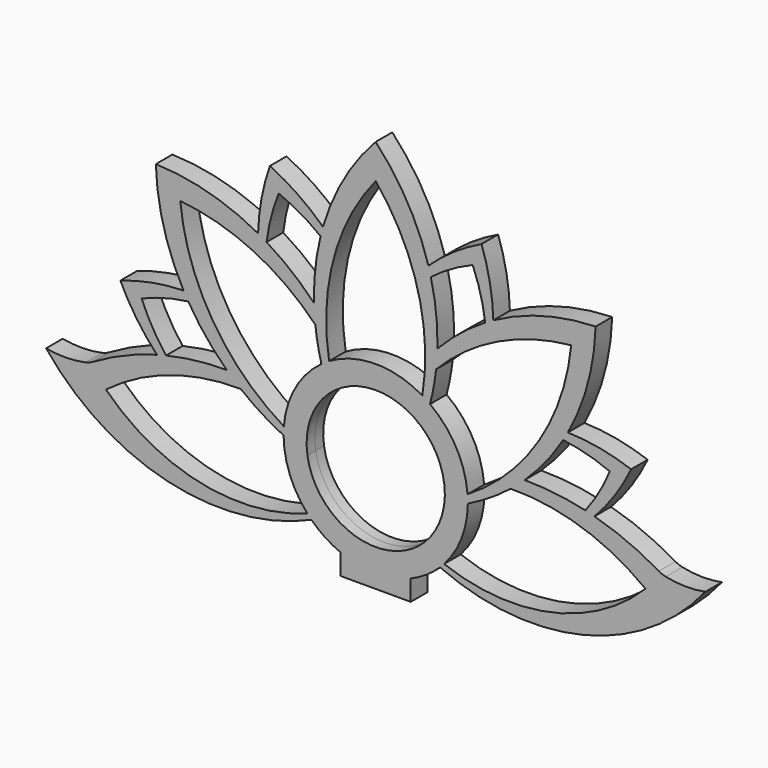
from build123d import *

# Parameters (mm, degrees)
F1_DEPTH = 4.5


# Not quite as in the source:
# - ends of sketch curves that miss each other by under 0.0002 mm in the source are joined


with BuildPart() as f1:
    # F0 (on Front) → F1 (new body, symmetric)
    with BuildSketch(Plane.XZ):
        with BuildLine():
            ThreePointArc((22.8784841202, 85.4427339913), (13.8060493669, 106.7545909747), (-1.20352e-05, 125.3528970532))
            ThreePointArc((-1.20352e-05, 125.3528970532), (-13.8060738367, 106.7545832167), (-22.8785085989, 85.4427260857))
            ThreePointArc((-22.8785085989, 85.4427260857), (-33.781429845, 94.2345199978), (-45.9220242093, 101.2184408782))
            ThreePointArc((-45.9220242093, 101.2184408782), (-49.5683429395, 87.6953665193), (-51.06114092, 73.7691058897))
            ThreePointArc((-51.06114092, 73.7691058897), (-72.5460800364, 82.4236845525), (-95.4594281867, 85.8123133595))
            ThreePointArc((-95.4594281867, 85.8123133595), (-92.0708001004, 62.8989646397), (-83.4162216453, 41.4140256538))
            ThreePointArc((-83.4162216453, 41.4140256538), (-97.3424818216, 39.9212276371), (-110.8655561911, 36.2749088727))
            ThreePointArc((-110.8655561911, 36.2749088727), (-103.8306945008, 24.0599857757), (-94.9659655862, 13.1005055314))
            ThreePointArc((-94.9659655862, 13.1005055314), (-109.3441086085, 8.1228594383), (-122.9337436667, 1.2796299938))
            ThreePointArc((-122.9337436667, 1.2796299938), (-124.3847743538, 0.5744976537), (-125.9303092338, 0.1118710562))
            ThreePointArc((-125.9303092338, 0.1118710562), (-134.5040813307, -0.8405705466), (-143.0970012567, -0.0800174007))
            ThreePointArc((-143.0970012567, -0.0800174007), (-90.2945054943, -33.7590284811), (-27.9154142382, -28.1707970164))
            ThreePointArc((-27.9154142382, -28.1707970164), (-21.9577774473, -32.956766848), (-15.1986970778, -36.5224048048))
            Line((-15.1986970778, -36.5224048048), (-15.1986972, -45.5224051023))
            Line((-15.1986972, -45.5224051023), (15.1986718, -45.5224051023))
            Line((15.1986718, -45.5224051023), (15.1986718, -36.5224051023))
            ThreePointArc((15.1986718, -36.5224051023), (21.9577523614, -32.9567672985), (27.9153889991, -28.1707973067))
            ThreePointArc((27.9153889991, -28.1707973067), (90.2944800943, -33.7590284811), (143.096975735, -0.0800170504))
            ThreePointArc((143.096975735, -0.0800170504), (134.5040559307, -0.8405705466), (125.9302837161, 0.1118705041))
            ThreePointArc((125.9302837161, 0.1118705041), (124.3847489538, 0.5744976537), (122.9337187314, 1.2796307814))
            ThreePointArc((122.9337187314, 1.2796307814), (109.3440836528, 8.1228592505), (94.9659404823, 13.1005047349))
            ThreePointArc((94.9659404823, 13.1005047349), (103.8306699794, 24.0599855987), (110.8655315962, 36.2749085192))
            ThreePointArc((110.8655315962, 36.2749085192), (97.3424564216, 39.9212276371), (83.416195792, 41.4140256177))
            ThreePointArc((83.416195792, 41.4140256177), (92.0707747004, 62.8989646397), (95.4594032906, 85.8123128836))
            ThreePointArc((95.4594032906, 85.8123128836), (72.5460546364, 82.4236845525), (51.0611157869, 73.7691059217))
            ThreePointArc((51.0611157869, 73.7691059217), (49.568318506, 87.695366698), (45.9219996628, 101.2184412045))
            ThreePointArc((45.9219996628, 101.2184412045), (33.7814018374, 94.2345137024), (22.8784841202, 85.4427339913))
        make_face()
        with BuildLine():
            ThreePointArc((-117.1095228717, -7.3640305351), (-89.448563488, 7.1418522166), (-58.5697361978, 11.837311045))
            ThreePointArc((-58.5697361978, 11.837311045), (-49.6119110254, 5.4631464022), (-39.9984925953, 0.1288430808))
            ThreePointArc((-39.9984925953, 0.1288430808), (-37.2748571799, -14.0339843315), (-29.705402075, -26.3102719896))
            ThreePointArc((-29.705402075, -26.3102719896), (-76.1944797379, -29.6944118928), (-117.1095228717, -7.3640305351))
        make_face(mode=Mode.SUBTRACT)
        with BuildLine():
            ThreePointArc((-91.0135912807, 14.1048128348), (-96.9513599422, 22.91124928), (-101.6267610462, 32.4480749604))
            ThreePointArc((-101.6267610462, 32.4480749604), (-91.6920273332, 35.8548732281), (-81.3873643524, 37.8844380956))
            ThreePointArc((-81.3873643524, 37.8844380956), (-73.7352473768, 26.9438563456), (-64.6715808547, 17.1407372042))
            ThreePointArc((-64.6715808547, 17.1407372042), (-77.9309186705, 16.3892197846), (-91.0135912807, 14.1048128348))
        make_face(mode=Mode.SUBTRACT)
        with BuildLine():
            ThreePointArc((-39.8747349061, 3.6409013815), (-70.812382671, 34.1134059196), (-84.8528261577, 75.2057109018))
            ThreePointArc((-84.8528261577, 75.2057109018), (-53.0294964681, 66.289674717), (-26.223286677, 46.9597204349))
            ThreePointArc((-26.223286677, 46.9597204349), (-25.1618451244, 39.8254262579), (-23.5802802502, 32.7881348844))
            ThreePointArc((-23.5802802502, 32.7881348844), (-34.9145400541, 19.9961948661), (-39.8747349061, 3.6409013815))
        make_face(mode=Mode.SUBTRACT)
        with BuildLine():
            ThreePointArc((58.569710798, 11.8373110298), (89.4485382345, 7.1418524965), (117.109497837, -7.3640300535))
            ThreePointArc((117.109497837, -7.3640300535), (76.1944543379, -29.6944118928), (29.7053768652, -26.3102719286))
            ThreePointArc((29.7053768652, -26.3102719286), (37.2748326568, -14.0339846476), (39.9984674303, 0.1288438922))
            ThreePointArc((39.9984674303, 0.1288438922), (49.6118856254, 5.4631464022), (58.569710798, 11.8373110298))
        make_face(mode=Mode.SUBTRACT)
        with BuildLine():
            ThreePointArc((-29.6372783208, -4.1734756121), (-2.3326090766, 30.3867739538), (29.9999878, 0.4775948977))
            ThreePointArc((29.9999878, 0.4775948977), (29.9091668501, -1.8550020562), (29.6372538967, -4.1734757653))
            ThreePointArc((29.6372538967, -4.1734757653), (-1.22775e-05, -29.5224051023), (-29.6372783208, -4.1734756121))
        make_face(mode=Mode.SUBTRACT)
        with BuildLine():
            ThreePointArc((26.2232617618, 46.9597209347), (53.0294713817, 66.2896748681), (84.8528008041, 75.2057108554))
            ThreePointArc((84.8528008041, 75.2057108554), (70.812357271, 34.1134059196), (39.8747095061, 3.6409013815))
            ThreePointArc((39.8747095061, 3.6409013815), (34.9145154377, 19.9961952532), (23.5802548967, 32.7881350301))
            ThreePointArc((23.5802548967, 32.7881350301), (25.161820701, 39.8254261326), (26.2232617618, 46.9597209347))
        make_face(mode=Mode.SUBTRACT)
        with BuildLine():
            ThreePointArc((81.3873389524, 37.8844380956), (91.6920019332, 35.8548732281), (101.6267360258, 32.4480754342))
            ThreePointArc((101.6267360258, 32.4480754342), (96.9513354477, 22.9112491166), (91.0135668807, 14.1048128348))
            ThreePointArc((91.0135668807, 14.1048128348), (77.930893754, 16.3892197289), (64.6715548016, 17.1407368356))
            ThreePointArc((64.6715548016, 17.1407368356), (73.7352219768, 26.9438563456), (81.3873389524, 37.8844380956))
        make_face(mode=Mode.SUBTRACT)
        with BuildLine():
            ThreePointArc((-47.3705884445, 71.6430268074), (-45.4199295453, 81.9895572502), (-42.0951898382, 91.9796457495))
            ThreePointArc((-42.0951898382, 91.9796457495), (-32.6613025725, 87.3636976735), (-23.9396864079, 81.5123196292))
            ThreePointArc((-23.9396864079, 81.5123196292), (-26.2649806939, 68.3652971805), (-26.7878526914, 55.0244649123))
            ThreePointArc((-26.7878526914, 55.0244649123), (-36.517789196, 64.0291013139), (-47.3705884445, 71.6430268074))
        make_face(mode=Mode.SUBTRACT)
        with BuildLine():
            ThreePointArc((-20.2364600157, 34.9810104129), (-18.2633780761, 74.8538230805), (-1.22419e-05, 110.352889417))
            ThreePointArc((-1.22419e-05, 110.352889417), (18.2633527585, 74.8538302889), (20.2364346157, 34.9810179281))
            ThreePointArc((20.2364346157, 34.9810179281), (-1.26313e-05, 40.4775948977), (-20.2364600157, 34.9810104129))
        make_face(mode=Mode.SUBTRACT)
        with BuildLine():
            ThreePointArc((23.9396582776, 81.5123130375), (32.6612744421, 87.3636910819), (42.0951621324, 91.9796391523))
            ThreePointArc((42.0951621324, 91.9796391523), (45.5019631468, 82.0449119699), (47.5315280138, 71.7402489249))
            ThreePointArc((47.5315280138, 71.7402489249), (36.5909469807, 64.0881318591), (26.7878276352, 55.0244650532))
            ThreePointArc((26.7878276352, 55.0244650532), (26.2649562826, 68.3652972858), (23.9396582776, 81.5123130375))
        make_face(mode=Mode.SUBTRACT)
    extrude(amount=F1_DEPTH, both=True)


solid = f1.part
